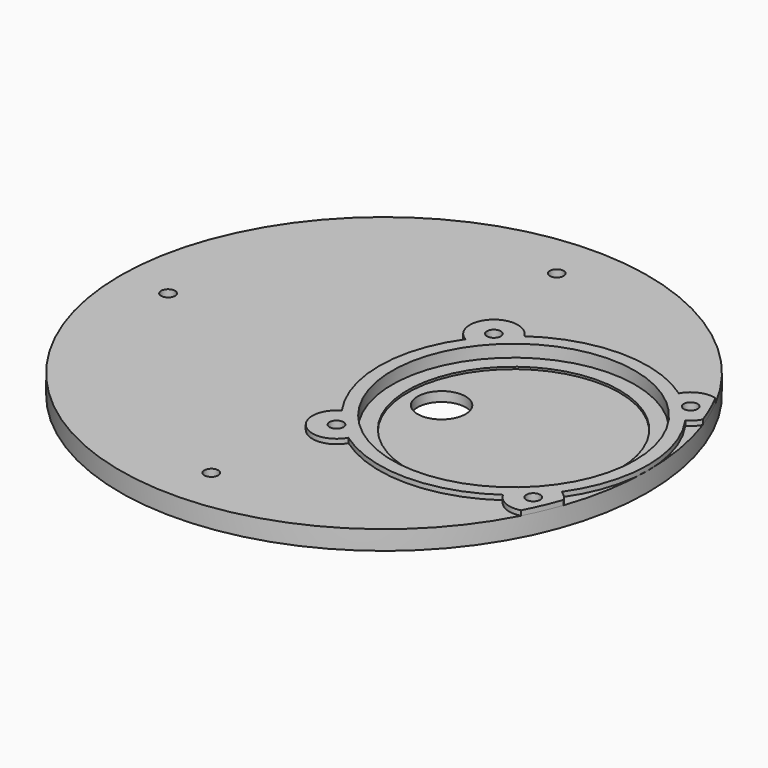
from build123d import *

# Parameters (mm, degrees)
F0_R      = 55
F1_DEPTH  = 4
F2_R      = 22.1
F3_DEPTH  = 2
F4_R      = 25.3
F4_R_2    = 22.1
F5_DEPTH  = 1.55
F6_R      = 28
F6_R_2    = 25.3
F7_DEPTH  = 1
F8_R      = 5
F9_DEPTH  = 25
F11_DEPTH = 1
F12_R     = 1.45
F13_DEPTH = 25
F14_R     = 1.45
F15_DEPTH = 25


with BuildPart() as f1:
    # F0 (on Top) → F1 (new body)
    with BuildSketch(Plane.XY):
        Circle(F0_R)
    extrude(amount=F1_DEPTH)

    # F2 (on face) → F3 (cut)
    with BuildSketch(Plane.XY.offset(4)):
        with Locations((27, 0)):
            Circle(F2_R)
    extrude(amount=-F3_DEPTH, mode=Mode.SUBTRACT)

    # F4 (on face) → F5 (cut)
    with BuildSketch(Plane.XY.offset(4)):
        with Locations((27, 0)):
            Circle(F4_R)
        with Locations((27, 0)):
            Circle(F4_R_2, mode=Mode.SUBTRACT)
    extrude(amount=-F5_DEPTH, mode=Mode.SUBTRACT)

    # F6 (on face) → F7 (join)
    with BuildSketch(Plane.XY.offset(4)):
        with Locations((27, 0)):
            Circle(F6_R)
        with Locations((27, 0)):
            Circle(F6_R_2, mode=Mode.SUBTRACT)
    extrude(amount=F7_DEPTH)

    # F8 (on face) → F9 (cut)
    with BuildSketch(Plane.XY.offset(2)):
        with Locations((12, 0)):
            Circle(F8_R)
    extrude(amount=-F9_DEPTH, mode=Mode.SUBTRACT)

    # F10 (on face) → F11 (join)
    with BuildSketch(Plane.XY.offset(4)):
        with BuildLine():
            ThreePointArc((10.8848586854, -22.8976466129), (7.2010101268, -19.7989898732), (4.1023533871, -16.1151413146))
            ThreePointArc((4.1023533871, -16.1151413146), (2.9583694397, -24.0416305603), (10.8848586854, -22.8976466129))
        make_face()
        with BuildLine():
            ThreePointArc((10.8848586854, 22.8976466129), (2.9583694397, 24.0416305603), (4.1023533871, 16.1151413146))
            ThreePointArc((4.1023533871, 16.1151413146), (7.2010101268, 19.7989898732), (10.8848586854, 22.8976466129))
        make_face()
        with BuildLine():
            ThreePointArc((49.8976466129, -16.1151413146), (46.7989898732, -19.7989898732), (43.1151413146, -22.8976466129))
            ThreePointArc((43.1151413146, -22.8976466129), (45.5447053375, -25.105329645), (48.8197581332, -25.3304404978))
            ThreePointArc((48.8197581332, -25.3304404978), (50.4964850216, -21.7969034605), (51.917853321, -18.1531404043))
            ThreePointArc((51.917853321, -18.1531404043), (51.0570972643, -16.9860974117), (49.8976466129, -16.1151413146))
        make_face()
        with BuildLine():
            ThreePointArc((48.8197581332, 25.3304404978), (45.5447053375, 25.105329645), (43.1151413146, 22.8976466129))
            ThreePointArc((43.1151413146, 22.8976466129), (46.7989898732, 19.7989898732), (49.8976466129, 16.1151413146))
            ThreePointArc((49.8976466129, 16.1151413146), (51.0570972643, 16.9860974117), (51.917853321, 18.1531404043))
            ThreePointArc((51.917853321, 18.1531404043), (50.4964850216, 21.7969034605), (48.8197581332, 25.3304404978))
        make_face()
    extrude(amount=F11_DEPTH)

    # F12 (on face) → F13 (cut)
    with BuildSketch(Plane.XY.offset(5)):
        with Locations((6.4939033456, 20.5060966544)):
            Circle(F12_R)
        with Locations((47.5060966544, 20.5060966544)):
            Circle(F12_R)
        with Locations((47.5060966544, -20.5060966544)):
            Circle(F12_R)
        with Locations((6.4939033456, -20.5060966544)):
            Circle(F12_R)
    extrude(amount=-F13_DEPTH, mode=Mode.SUBTRACT)

    # F14 (on face) → F15 (cut)
    with BuildSketch(Plane.XY.offset(4)):
        with Locations((0, 45)):
            Circle(F14_R)
        with Locations((-45, 0)):
            Circle(F14_R)
        with Locations((0, -45)):
            Circle(F14_R)
    extrude(amount=-F15_DEPTH, mode=Mode.SUBTRACT)


solid = f1.part
